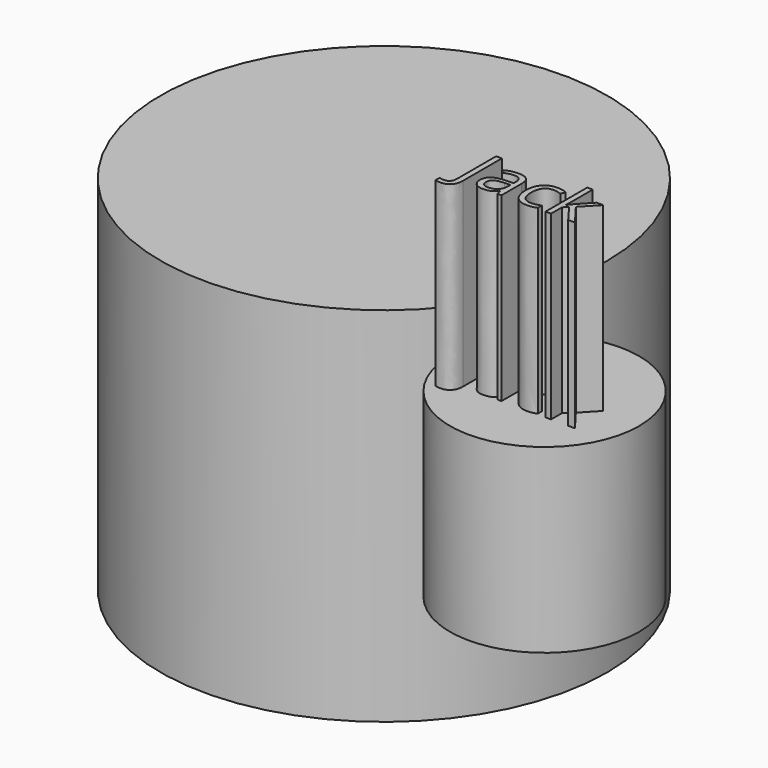
from build123d import *

# Parameters (mm, degrees)
F0_R         = 31.3290670099
F1_DEPTH     = 25.4
F3_DEPTH     = 25.4
F4_R         = 13.2654631177
F5_DEPTH     = 25.4
F6_TEXT_SIZE = 9.6085533086
F7_DEPTH     = 25.4


# Not quite as in the source:
# - Text() gives the source's letters only with a copy of the font that has no kerning and outlines rounded to 1/6400 em; it was checked with that copy


with BuildPart() as f1:
    # F0 (on Top) → F1 (new body)
    with BuildSketch(Plane.XY):
        Circle(F0_R)
    extrude(amount=F1_DEPTH)

    # F3 (add): a face of the model
    f3_faces = [f1.faces().sort_by_distance(p)[0] for p in [
        (0, 0, 0),
    ]]
    extrude(f3_faces, amount=F3_DEPTH)


with BuildPart() as f5:
    # F4 (on Top) → F5 (new body)
    with BuildSketch(Plane.XY):
        with Locations((45.2688150108, -28.4246038646)):
            Circle(F4_R)
    extrude(amount=F5_DEPTH)

    # F6 (on face) → F7 (join)
    with BuildSketch(Plane.XY.offset(25.4)):
        with Locations((35.9443463385, -33.2372374833)):
            Text('Jack', F6_TEXT_SIZE, font='Open Sans', text_align=(TextAlign.LEFT, TextAlign.BOTTOM))
    extrude(amount=F7_DEPTH)


solid = Compound([f1.part, f5.part])
